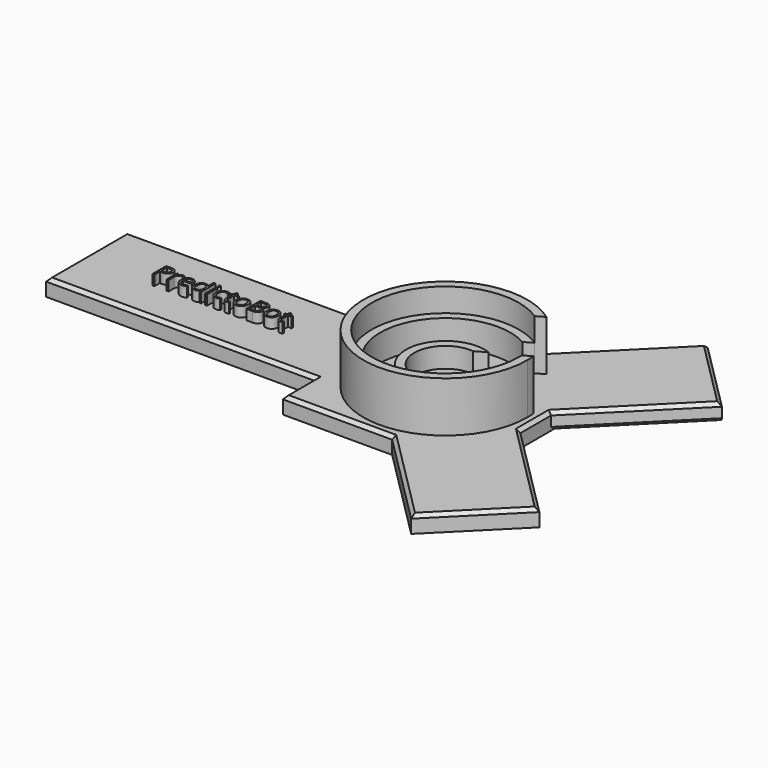
from build123d import *

# Parameters (mm, degrees)
F0_W         = 80
F0_H         = 30
F1_DEPTH     = 5
F3_DEPTH     = 15
F4_DEPTH     = 8
F5_SIZE      = 1
F6_DEPTH     = 6
F7_TEXT_SIZE = 7.2474025423
F8_DEPTH     = 3


# Not quite as in the source:
# - Text() gives the source's letters only with a copy of the font that has no kerning and outlines rounded to 1/6400 em; it was checked with that copy


with BuildPart() as f1:
    # F0 (on Top) → F1 (new body)
    with BuildSketch(Plane.XY):
        Polygon((26.9, -5.69), (26.9, -26.9), (5.69, -26.9), (33.9742712475, -55.1842712475), (55.1842712475, -33.9742712475), align=None)
        Polygon((5.69, -26.9), (26.9, -26.9), (26.9, -5.69), (26.9, 5.69), (26.9, 26.9), (5.69, 26.9), (-26.9, 26.9), (-26.9, 15), (-26.9, -15), (-26.9, -26.9), align=None)
        Polygon((26.9, 26.9), (26.9, 5.69), (55.1842712475, 33.9742712475), (33.9742712475, 55.1842712475), (5.69, 26.9), align=None)
        with Locations((-66.9, 0)):
            Rectangle(F0_W, F0_H)
    extrude(amount=F1_DEPTH)

    # F2 (on face) → F3 (join)
    with BuildSketch(Plane.XY.offset(5)):
        with BuildLine():
            ThreePointArc((21.8732776899, 1.0815373785), (21.8933184032, 0.5409337258), (21.9, 0))
            ThreePointArc((21.9, 0), (-19.2306367732, -10.4781968533), (11.8732776899, 18.4020454542))
            Line((11.8732776899, 18.4020454542), (14.2748540851, 19.7885962324))
            ThreePointArc((14.2748540851, 19.7885962324), (-21.7217223037, -11.1142602166), (24.4, 0))
            ThreePointArc((24.4, 0), (24.3686934372, 1.23562946), (24.2748540851, 2.4680881568))
            Line((24.2748540851, 2.4680881568), (21.8732776899, 1.0815373785))
        make_face()
    extrude(amount=F3_DEPTH)

    # F2 (on face) → F4 (join)
    with BuildSketch(Plane.XY.offset(5)):
        with BuildLine():
            ThreePointArc((11.8732776899, 18.4020454542), (-19.2306367732, -10.4781968533), (21.9, 0))
            ThreePointArc((21.9, 0), (21.8933184032, 0.5409337258), (21.8732776899, 1.0815373785))
            Line((21.8732776899, 1.0815373785), (19.3968746608, -0.3482145769))
            ThreePointArc((19.3968746608, -0.3482145769), (-16.8008928334, -9.7), (9.3968746608, 16.9722934988))
            Line((9.3968746608, 16.9722934988), (11.8732776899, 18.4020454542))
        make_face()
    extrude(amount=F4_DEPTH)

    # F5
    f5_edges = [f1.edges().sort_by_distance(p)[0] for p in [
        (-66.9, -15, 5),
        (-106.9, 0, 5),
        (-66.9, 15, 5),
        (-26.9, -20.95, 5),
        (-10.605, -26.9, 5),
        (19.832136, -41.042136, 5),
        (44.579271, -44.579271, 5),
        (41.042136, -19.832136, 5),
        (41.042136, 19.832136, 0),
        (19.832136, 41.042136, 5),
        (-10.605, 26.9, 5),
        (-26.9, 20.95, 5),
        (26.9, 0, 5),
        (44.579271, 44.579271, 5),
        (41.042136, 19.832136, 5),
    ]]
    chamfer(f5_edges, length=F5_SIZE)

    # F2 (on face) → F6 (join)
    with BuildSketch(Plane.XY.offset(5)):
        with BuildLine():
            Line((0.9387498334, 9.2022415068), (4.0832225169, 11.0177036572))
            ThreePointArc((4.0832225169, 11.0177036572), (-10.1757984945, -5.875), (11.5832225169, -1.9726773996))
            Line((11.5832225169, -1.9726773996), (8.4387498334, -3.7881395499))
            ThreePointArc((8.4387498334, -3.7881395499), (-8.010734985, -4.625), (0.9387498334, 9.2022415068))
        make_face()
    extrude(amount=F6_DEPTH)

    # F7 (on face) → F8 (join)
    with BuildSketch(Plane.XY.offset(5)):
        with Locations((-85.9, -2.6091298304)):
            Text('PredictoBot', F7_TEXT_SIZE, font='Open Sans', text_align=(TextAlign.LEFT, TextAlign.BOTTOM))
    extrude(amount=F8_DEPTH)


solid = f1.part
